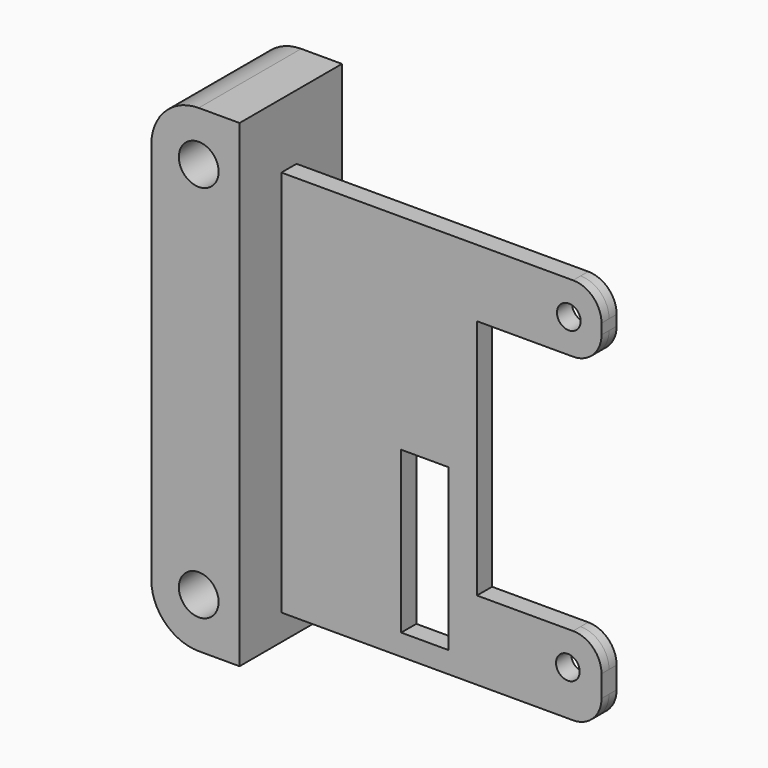
from build123d import *

# Parameters (mm, degrees)
F0_R          = 2.667
F0_R_2        = 1.5875
F0_W          = 6.35
F0_H          = 21.59
F1_DEPTH      = 1.27
F2_R          = 2.667
F3_DEPTH      = 7.62
F3_DEPTH_BACK = 9.5504
F4_TEXT_SIZE  = 28.8275341028
F5_DEPTH      = 1.524
F7_DEPTH      = 25.4
F8_R          = 3.81
F9_W          = 6.35
F9_H          = 21.59
F9_R          = 1.5875
F10_DEPTH     = 1.27


# Not quite as in the source:
# - a feature names something its author has since deleted; it is built from what else it names
# - Text() gives the source's letters only with a copy of the font that has no kerning and outlines rounded to 1/6400 em; it was checked with that copy


with BuildPart() as f1:
    # F0 (on Front) → F1 (new body)
    with BuildSketch(Plane.XZ):
        with BuildLine():
            Line((-85.725, 0), (-136.525, 0))
            ThreePointArc((-136.525, 0), (-141.0151280605, -1.8598719395), (-142.875, -6.35))
            Line((-142.875, -6.35), (-142.875, -57.785))
            ThreePointArc((-142.875, -57.785), (-141.0151280605, -62.2751280605), (-136.525, -64.135))
            Line((-136.525, -64.135), (-85.725, -64.135))
            Line((-85.725, -64.135), (-85.725, 0))
        make_face()
        with Locations((-136.525, -57.4675)):
            Circle(F0_R, mode=Mode.SUBTRACT)
        with Locations((-92.630498, -54.61)):
            Circle(F0_R_2, mode=Mode.SUBTRACT)
        with Locations((-111.807625, -46.99)):
            Rectangle(F0_W, F0_H, mode=Mode.SUBTRACT)
        with Locations((-136.525, -6.6675)):
            Circle(F0_R, mode=Mode.SUBTRACT)
        with Locations((-92.503498, -13.208)):
            Circle(F0_R_2, mode=Mode.SUBTRACT)
    extrude(amount=F1_DEPTH)

    # F2 (on face) → F3 (join, two sides)
    with BuildSketch(Plane(origin=(0, 0, 0), x_dir=(-1, 0, 0), z_dir=(0, 1, 0))) as f3_sk:
        with BuildLine():
            Line((131.047998, 0), (131.047998, -64.135))
            Line((131.047998, -64.135), (136.525, -64.135))
            ThreePointArc((136.525, -64.135), (141.0151280605, -62.2751280605), (142.875, -57.785))
            Line((142.875, -57.785), (142.875, -6.35))
            ThreePointArc((142.875, -6.35), (141.0151280605, -1.8598719395), (136.525, 0))
            Line((136.525, 0), (131.047998, 0))
        make_face()
        with Locations((136.525, -57.4675)):
            Circle(F2_R, mode=Mode.SUBTRACT)
        with Locations((136.525, -6.6675)):
            Circle(F2_R, mode=Mode.SUBTRACT)
    extrude(amount=F3_DEPTH)
    extrude(f3_sk.sketch, amount=-F3_DEPTH_BACK)

    # F4 (on face) → F5 (cut)
    with BuildSketch(Plane(origin=(-142.875, 0, 0), x_dir=(0, -1, 0), z_dir=(-1, 0, 0))):
        with Locations((-7.62, -41.8095169326)):
            Text('L', F4_TEXT_SIZE, font='Open Sans', font_style=FontStyle.BOLD, text_align=(TextAlign.LEFT, TextAlign.BOTTOM))
    extrude(amount=-F5_DEPTH, mode=Mode.SUBTRACT)

    # F6 (on face) → F7 (cut)
    with BuildSketch(Plane.XZ.offset(1.27)):
        Polygon((-85.725, 0), (-131.047998, 0), (-131.047998, -8.6995), (-88.121998, -8.6995), (-88.121998, -17.7165), (-104.822625, -17.7165), (-104.822625, -50.1015), (-88.121998, -50.1015), (-88.121998, -60.6425), (-131.047998, -60.6425), (-131.047998, -64.135), (-85.725, -64.135), align=None)
    extrude(amount=-F7_DEPTH, mode=Mode.SUBTRACT)

    # F8
    f8_edges = [f1.edges().sort_by_distance(p)[0] for p in [
        (-88.121998, -0.635, -8.6995),
        (-88.121998, -0.635, -50.1015),
        (-88.121998, -0.635, -60.6425),
        (-88.121998, -0.635, -17.7165),
    ]]
    fillet(f8_edges, radius=F8_R)

    # F9 (on face) → F10 (join)
    with BuildSketch(Plane.XZ.offset(1.27)):
        with BuildLine():
            Line((-91.931998, -8.6995), (-131.047998, -8.6995))
            Line((-131.047998, -8.6995), (-131.047998, -60.6425))
            Line((-131.047998, -60.6425), (-91.931998, -60.6425))
            ThreePointArc((-91.931998, -60.6425), (-89.2379211637, -59.5265768363), (-88.121998, -56.8325))
            Line((-88.121998, -56.8325), (-88.121998, -53.9115))
            ThreePointArc((-88.121998, -53.9115), (-89.2379211637, -51.2174231637), (-91.931998, -50.1015))
            Line((-91.931998, -50.1015), (-104.822625, -50.1015))
            Line((-104.822625, -50.1015), (-104.822625, -17.7165))
            Line((-104.822625, -17.7165), (-91.931998, -17.7165))
            ThreePointArc((-91.931998, -17.7165), (-89.2379211637, -16.6005768363), (-88.121998, -13.9065))
            Line((-88.121998, -13.9065), (-88.121998, -12.5095))
            ThreePointArc((-88.121998, -12.5095), (-89.2379211637, -9.8154231637), (-91.931998, -8.6995))
        make_face()
        with Locations((-111.807625, -46.99)):
            Rectangle(F9_W, F9_H, mode=Mode.SUBTRACT)
        with Locations((-92.630498, -54.61)):
            Circle(F9_R, mode=Mode.SUBTRACT)
        with Locations((-92.503498, -13.208)):
            Circle(F9_R, mode=Mode.SUBTRACT)
    extrude(amount=F10_DEPTH)


solid = f1.part
